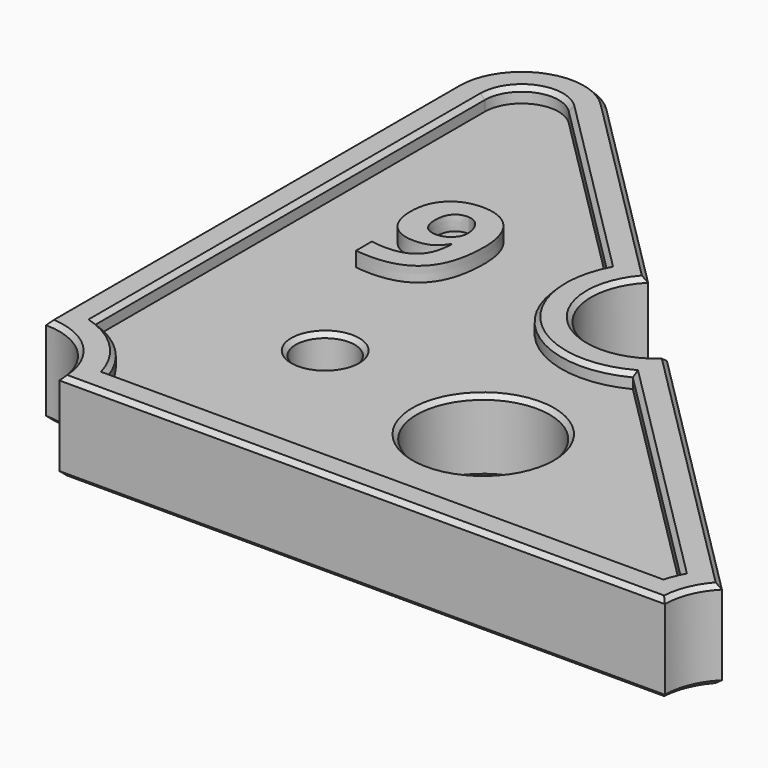
from build123d import *

# Parameters (mm, degrees)
F0_R         = 2
F0_R_2       = 4.5
F0_TEXT_SIZE = 11.1111111111
F1_DEPTH     = 5
F3_DEPTH     = 1
F4_SIZE      = 0.3


# Not quite as in the source:
# - Text() gives the source's letters only with a copy of the font that has no kerning and outlines rounded to 1/6400 em; it was checked with that copy


with BuildPart() as f1:
    # F0 (on Top) → F1 (new body)
    with BuildSketch(Plane.XY):
        with BuildLine():
            ThreePointArc((-17.3180194847, 17.3180194847), (-22.2220754456, 18.2934968656), (-25, 14.1360389693))
            Line((-25, 14.1360389693), (-25, -20.5))
            ThreePointArc((-25, -20.5), (-21.8180194847, -21.8180194847), (-20.5, -25))
            Line((-20.5, -25), (20.5, -25))
            ThreePointArc((20.5, -25), (20.8425421037, -23.2779245544), (21.8180194847, -21.8180194847))
            Line((21.8180194847, -21.8180194847), (3.1819805153, -3.1819805153))
            ThreePointArc((3.1819805153, -3.1819805153), (-3.1819805153, -3.1819805153), (-3.1819805153, 3.1819805153))
            Line((-3.1819805153, 3.1819805153), (-17.3180194847, 17.3180194847))
        make_face()
        with Locations((-12.5, -12.5)):
            Circle(F0_R, mode=Mode.SUBTRACT)
        with Locations((0, -14.75)):
            Circle(F0_R_2, mode=Mode.SUBTRACT)
        with BuildLine():
            add(Edge.make_bspline(
                [(-12.484375, 2.4157986111), (-12.1319444444, 1.6319444444), (-12.1319444444, 0.546875)],
                knots=[0, 0, 0, 1, 1, 1], degree=2))
            add(Edge.make_bspline(
                [(-12.1319444444, 0.546875), (-12.1319444444, -1.796875), (-13.1189236111, -2.953125)],
                knots=[0, 0, 0, 1, 1, 1], degree=2))
            add(Edge.make_bspline(
                [(-13.1189236111, -2.953125), (-14.1059027778, -4.109375), (-16.1076388889, -4.109375)],
                knots=[0, 0, 0, 1, 1, 1], degree=2))
            add(Edge.make_bspline(
                [(-16.1076388889, -4.109375), (-16.8142361111, -4.109375), (-17.1770833333, -4.0329861111)],
                knots=[0, 0, 0, 1, 1, 1], degree=2))
            Line((-17.1770833333, -4.0329861111), (-17.1770833333, -2.6875))
            add(Edge.make_bspline(
                [(-17.1770833333, -2.6875), (-16.7204861111, -2.8003472222), (-16.2222222222, -2.8003472222)],
                knots=[0, 0, 0, 1, 1, 1], degree=2))
            add(Edge.make_bspline(
                [(-16.2222222222, -2.8003472222), (-15.3819444444, -2.8003472222), (-14.8394097222, -2.5538194444)],
                knots=[0, 0, 0, 1, 1, 1], degree=2))
            add(Edge.make_bspline(
                [(-14.8394097222, -2.5538194444), (-14.296875, -2.3072916667), (-14.0086805556, -1.7786458333)],
                knots=[0, 0, 0, 1, 1, 1], degree=2))
            add(Edge.make_bspline(
                [(-14.0086805556, -1.7786458333), (-13.7204861111, -1.25), (-13.6770833333, -0.3211805556)],
                knots=[0, 0, 0, 1, 1, 1], degree=2))
            Line((-13.6770833333, -0.3211805556), (-13.7430555556, -0.3211805556))
            add(Edge.make_bspline(
                [(-13.7430555556, -0.3211805556), (-14.0572916667, -0.8315972222), (-14.4696180556, -1.0373263889)],
                knots=[0, 0, 0, 1, 1, 1], degree=2))
            add(Edge.make_bspline(
                [(-14.4696180556, -1.0373263889), (-14.8819444444, -1.2430555556), (-15.5, -1.2430555556)],
                knots=[0, 0, 0, 1, 1, 1], degree=2))
            add(Edge.make_bspline(
                [(-15.5, -1.2430555556), (-16.5364583333, -1.2430555556), (-17.1336805556, -0.5789930556)],
                knots=[0, 0, 0, 1, 1, 1], degree=2))
            add(Edge.make_bspline(
                [(-17.1336805556, -0.5789930556), (-17.7309027778, 0.0850694444), (-17.7309027778, 1.2673611111)],
                knots=[0, 0, 0, 1, 1, 1], degree=2))
            add(Edge.make_bspline(
                [(-17.7309027778, 1.2673611111), (-17.7309027778, 2.5434027778), (-17.0060763889, 3.2838541667)],
                knots=[0, 0, 0, 1, 1, 1], degree=2))
            add(Edge.make_bspline(
                [(-17.0060763889, 3.2838541667), (-16.28125, 4.0243055556), (-15.0347222222, 4.0243055556)],
                knots=[0, 0, 0, 1, 1, 1], degree=2))
            add(Edge.make_bspline(
                [(-15.0347222222, 4.0243055556), (-14.1545138889, 4.0243055556), (-13.4956597222, 3.6119791667)],
                knots=[0, 0, 0, 1, 1, 1], degree=2))
            add(Edge.make_bspline(
                [(-13.4956597222, 3.6119791667), (-12.8368055556, 3.1996527778), (-12.484375, 2.4157986111)],
                knots=[0, 0, 0, 1, 1, 1], degree=2))
        make_face(mode=Mode.SUBTRACT)
        with Locations((-18.0885416667, -4)):
            Text('9', F0_TEXT_SIZE, font='Open Sans', font_style=FontStyle.BOLD, text_align=(TextAlign.LEFT, TextAlign.BOTTOM))
        with BuildLine():
            add(Edge.make_bspline(
                [(-14.1362847222, 2.2335069444), (-14.4756944444, 2.6788194444), (-15.0017361111, 2.6788194444)],
                knots=[0, 0, 0, 1, 1, 1], degree=2))
            add(Edge.make_bspline(
                [(-15.0017361111, 2.6788194444), (-15.5225694444, 2.6788194444), (-15.8151041667, 2.3203125)],
                knots=[0, 0, 0, 1, 1, 1], degree=2))
            add(Edge.make_bspline(
                [(-15.8151041667, 2.3203125), (-16.1076388889, 1.9618055556), (-16.1076388889, 1.2899305556)],
                knots=[0, 0, 0, 1, 1, 1], degree=2))
            add(Edge.make_bspline(
                [(-16.1076388889, 1.2899305556), (-16.1076388889, 0.7152777778), (-15.8420138889, 0.3784722222)],
                knots=[0, 0, 0, 1, 1, 1], degree=2))
            add(Edge.make_bspline(
                [(-15.8420138889, 0.3784722222), (-15.5763888889, 0.0416666667), (-15.0347222222, 0.0416666667)],
                knots=[0, 0, 0, 1, 1, 1], degree=2))
            add(Edge.make_bspline(
                [(-15.0347222222, 0.0416666667), (-14.5243055556, 0.0416666667), (-14.1605902778, 0.3758680556)],
                knots=[0, 0, 0, 1, 1, 1], degree=2))
            add(Edge.make_bspline(
                [(-14.1605902778, 0.3758680556), (-13.796875, 0.7100694444), (-13.796875, 1.1440972222)],
                knots=[0, 0, 0, 1, 1, 1], degree=2))
            add(Edge.make_bspline(
                [(-13.796875, 1.1440972222), (-13.796875, 1.7881944444), (-14.1362847222, 2.2335069444)],
                knots=[0, 0, 0, 1, 1, 1], degree=2))
        make_face()
    extrude(amount=-F1_DEPTH)

    # F0 (on Top) + F2 (on face) → F3 (join)
    with BuildSketch(Plane.XY):
        with Locations((-18.0885416667, -4)):
            Text('9', F0_TEXT_SIZE, font='Open Sans', font_style=FontStyle.BOLD, text_align=(TextAlign.LEFT, TextAlign.BOTTOM))
    with BuildSketch(Plane.XY):
        with BuildLine():
            ThreePointArc((20.5, -25), (20.8425421037, -23.2779245544), (21.8180194847, -21.8180194847))
            Line((21.8180194847, -21.8180194847), (3.1819805153, -3.1819805153))
            ThreePointArc((3.1819805153, -3.1819805153), (-3.1819805153, -3.1819805153), (-3.1819805153, 3.1819805153))
            Line((-3.1819805153, 3.1819805153), (-17.3180194847, 17.3180194847))
            ThreePointArc((-17.3180194847, 17.3180194847), (-22.2220754456, 18.2934968656), (-25, 14.1360389693))
            Line((-25, 14.1360389693), (-25, -20.5))
            ThreePointArc((-25, -20.5), (-21.8180194847, -21.8180194847), (-20.5, -25))
            Line((-20.5, -25), (20.5, -25))
        make_face()
        with BuildLine():
            Line((2.9590003588, -5.7874274835), (19.2125725165, -22.0409996412))
            ThreePointArc((19.2125725165, -22.0409996412), (18.9947830387, -22.5125576896), (18.8153415616, -23))
            Line((18.8153415616, -23), (-18.8153415616, -23))
            ThreePointArc((-18.8153415616, -23), (-20.4038059223, -20.4038059223), (-23, -18.8153415616))
            Line((-23, -18.8153415616), (-23, 14.1360389693))
            ThreePointArc((-23, 14.1360389693), (-21.4567085809, 16.4457378006), (-18.732233047, 15.9038059223))
            Line((-18.732233047, 15.9038059223), (-5.7874274835, 2.9590003588))
            ThreePointArc((-5.7874274835, 2.9590003588), (-4.5961940777, -4.5961940777), (2.9590003588, -5.7874274835))
        make_face(mode=Mode.SUBTRACT)
    extrude(amount=F3_DEPTH)

    # F4
    f4_edges = [f1.edges().sort_by_distance(p)[0] for p in [
        (-14.5, -12.5, 0),
        (-4.5, -14.75, 0),
        (-21.818019, -21.818019, 1),
        (0, -25, 1),
        (20.842542, -23.277925, 1),
        (12.5, -12.5, 1),
        (-3.181981, -3.181981, 1),
        (-10.25, 10.25, 1),
        (-22.222075, 18.293497, 1),
        (-25, -3.181981, 1),
        (-12.25983, 9.431403, 1),
        (-4.596194, -4.596194, 1),
        (11.085786, -13.914214, 1),
        (18.994783, -22.512558, 1),
        (0, -23, 1),
        (-20.403806, -20.403806, 1),
        (-23, -2.339651, 1),
        (-21.456709, 16.445738, 1),
        (12.5, -12.5, -5),
        (-3.181981, -3.181981, -5),
        (-10.25, 10.25, -5),
        (-22.222075, 18.293497, -5),
        (-25, -3.181981, -5),
        (-21.818019, -21.818019, -5),
        (0, -25, -5),
        (20.842542, -23.277925, -5),
        (-14.5, -12.5, -5),
        (-4.5, -14.75, -5),
    ]]
    chamfer(f4_edges, length=F4_SIZE)


solid = f1.part
